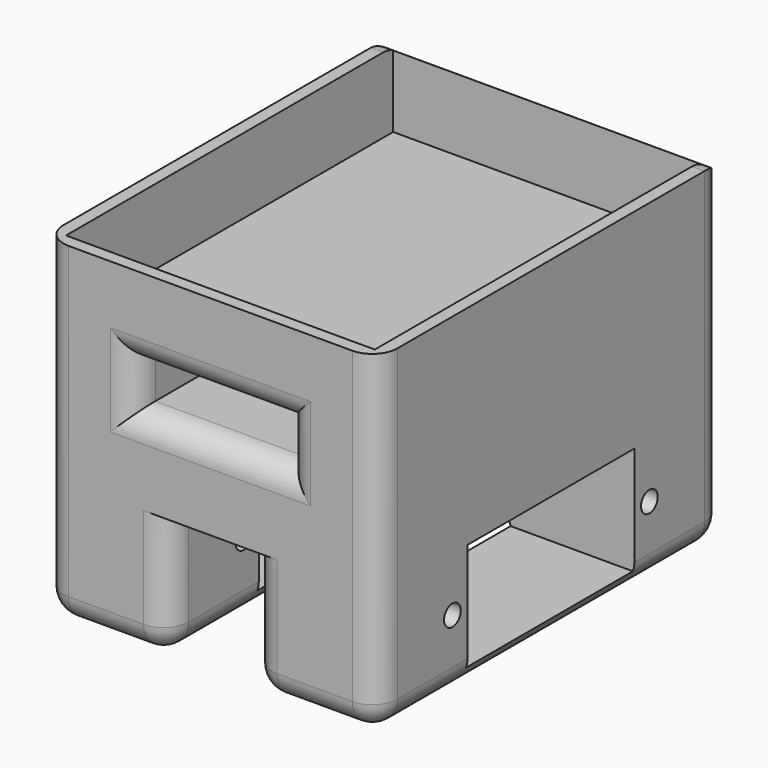
from build123d import *

# Parameters (mm, degrees)
F0_W           = 40
F0_H           = 52
F1_DEPTH       = 40
F2_W           = 25
F2_H           = 13
F2_R           = 1.25
F3_DEPTH       = 40.001
F4_W           = 10
F4_H           = 52
F5_DEPTH       = 15
F6_W           = 25
F6_H           = 6
F7_DEPTH       = 42
F8_W           = 18
F8_H           = 5
F9_DEPTH       = 42
F10_W          = 37
F10_H          = 49
F11_DEPTH      = 9
F12_T1_DEPTH   = 37
F12_T3_DEPTH   = 25
F12_T5_DEPTH   = 9
F12_T7_DEPTH   = 12
F12_T9_DEPTH   = 40
F12_T11_DEPTH  = 10
F12_T13_DEPTH  = 9
F12_T15_DEPTH  = 6
F12_T17_DEPTH  = 5
F12_T19_DEPTH  = 18
F12_T21_DEPTH  = 46
F12_S25_W      = 3.06
F12_S25_H      = 3.06
F12_T26_DEPTH  = 3.06
F12_S31_W      = 3.06
F12_S31_H      = 3.06
F12_T32_DEPTH  = 3.06
F12_S37_W      = 3.06
F12_S37_H      = 3.06
F12_T38_DEPTH  = 3.06
F12_S43_W      = 3.06
F12_S43_H      = 3.06
F12_T44_DEPTH  = 3.06
F12_S49_W      = 3.06
F12_S49_H      = 3.06
F12_T50_DEPTH  = 3.06
F12_S55_W      = 3.06
F12_S55_H      = 3.06
F12_T56_DEPTH  = 3.06
F12_S61_W      = 3.06
F12_S61_H      = 3.06
F12_T62_DEPTH  = 3.06
F12_S67_W      = 3.06
F12_S67_H      = 3.06
F12_T68_DEPTH  = 3.06
F12_T75_DEPTH  = 47.5
F12_T79_DEPTH  = 44.5
F12_T86_DEPTH  = 44.5
F12_T90_DEPTH  = 47.5
F12_T97_DEPTH  = 32.5
F12_T101_DEPTH = 13.5
F12_T108_DEPTH = 13.5
F12_T112_DEPTH = 32.5
F12_T119_DEPTH = 19.5
F12_T123_DEPTH = 17.5
F12_T130_DEPTH = 17.5
F12_T134_DEPTH = 19.5
F12_T141_DEPTH = 13.5
F12_T145_DEPTH = 32.5
F12_T152_DEPTH = 13.5
F12_T156_DEPTH = 32.5
F12_T163_DEPTH = 12.5
F12_T167_DEPTH = 25.5
F12_T174_DEPTH = 25.5
F12_T178_DEPTH = 12.5
F12_T185_DEPTH = 12.5
F12_T189_DEPTH = 25.5
F12_T196_DEPTH = 12.5
F12_T200_DEPTH = 25.5


# Not quite as in the source:
# - a fillet or chamfer that OpenCascade refuses, or shapes differently, is made with other operations: its cross-section is extruded or revolved along the edge and cut away or added


with BuildPart() as f1:
    # F0 (on Top) → F1 (new body)
    with BuildSketch(Plane.XY):
        with Locations((9.9251037464, 5.5336094776)):
            Rectangle(F0_W, F0_H)
    extrude(amount=F1_DEPTH)

    # F2 (on face) → F3 (cut, through all)
    with BuildSketch(Plane.YZ.offset(29.9251037464)):
        with Locations((5.5336094776, 8.5)):
            Rectangle(F2_W, F2_H)
        with Locations((-9.2163905224, 8.5)):
            Circle(F2_R)
        with Locations((20.2836094776, 8.5)):
            Circle(F2_R)
    extrude(amount=-F3_DEPTH, mode=Mode.SUBTRACT)

    # F4 (on face) → F5 (cut)
    with BuildSketch(Plane(origin=(0, 0, 0), x_dir=(1, 0, 0), z_dir=(0, 0, -1))):
        with Locations((9.9251037464, -5.5336094776)):
            Rectangle(F4_W, F4_H)
    extrude(amount=-F5_DEPTH, mode=Mode.SUBTRACT)

    # F6 (on face) → F7 (cut)
    with BuildSketch(Plane(origin=(0, 31.5336094776, 0), x_dir=(-1, 0, 0), z_dir=(0, 1, 0))):
        with Locations((-9.9251037464, 20)):
            Rectangle(F6_W, F6_H)
    extrude(amount=-F7_DEPTH, mode=Mode.SUBTRACT)

    # F8 (on face) → F9 (cut)
    with BuildSketch(Plane.XZ.offset(20.4663905224)):
        with Locations((9.9251037464, 27.5)):
            Rectangle(F8_W, F8_H)
    extrude(amount=-F9_DEPTH, mode=Mode.SUBTRACT)

    # F10 (on face) → F11 (cut)
    with BuildSketch(Plane.XY.offset(40)):
        with Locations((9.9251037464, 5.5336094776)):
            Rectangle(F10_W, F10_H)
    extrude(amount=-F11_DEPTH, mode=Mode.SUBTRACT)

    # F12: fillet of radius 3 on 26 edges, made by hand

    # F12_s2 → F12_t1 (cut)
    with BuildSketch(Plane.XY.offset(3)):
        with BuildLine():
            ThreePointArc((-10.0748962536, -17.4663905224), (-9.1962165972, -19.587710866), (-7.0748962536, -20.4663905224))
            Line((-7.0748962536, -20.4663905224), (-7.0748962536, -20.5263905224))
            Line((-7.0748962536, -20.5263905224), (-10.1348962536, -20.5263905224))
            Line((-10.1348962536, -20.5263905224), (-10.1348962536, -17.4663905224))
            Line((-10.1348962536, -17.4663905224), (-10.0748962536, -17.4663905224))
        make_face()
        with BuildLine():
            ThreePointArc((29.9251037464, -17.4663905224), (29.0464240899, -19.587710866), (26.9251037464, -20.4663905224))
            Line((26.9251037464, -20.4663905224), (26.9251037464, -20.5263905224))
            Line((26.9251037464, -20.5263905224), (29.9851037464, -20.5263905224))
            Line((29.9851037464, -20.5263905224), (29.9851037464, -17.4663905224))
            Line((29.9851037464, -17.4663905224), (29.9251037464, -17.4663905224))
        make_face()
        with BuildLine():
            ThreePointArc((-7.0748962536, 31.5336094776), (-9.1962165972, 30.6549298212), (-10.0748962536, 28.5336094776))
            Line((-10.0748962536, 28.5336094776), (-10.1348962536, 28.5336094776))
            Line((-10.1348962536, 28.5336094776), (-10.1348962536, 31.5936094776))
            Line((-10.1348962536, 31.5936094776), (-7.0748962536, 31.5936094776))
            Line((-7.0748962536, 31.5936094776), (-7.0748962536, 31.5336094776))
        make_face()
        with BuildLine():
            ThreePointArc((26.9251037464, 31.5336094776), (29.0464240899, 30.6549298212), (29.9251037464, 28.5336094776))
            Line((29.9251037464, 28.5336094776), (29.9851037464, 28.5336094776))
            Line((29.9851037464, 28.5336094776), (29.9851037464, 31.5936094776))
            Line((29.9851037464, 31.5936094776), (26.9251037464, 31.5936094776))
            Line((26.9251037464, 31.5936094776), (26.9251037464, 31.5336094776))
        make_face()
    extrude(amount=F12_T1_DEPTH, mode=Mode.SUBTRACT)

    # F12_s4 → F12_t3 (cut)
    with BuildSketch(Plane.YZ.offset(-2.5748962536)):
        with BuildLine():
            ThreePointArc((31.5336094776, 14), (30.6549298212, 16.1213203436), (28.5336094776, 17))
            Line((28.5336094776, 17), (28.5336094776, 17.06))
            Line((28.5336094776, 17.06), (31.5936094776, 17.06))
            Line((31.5936094776, 17.06), (31.5936094776, 14))
            Line((31.5936094776, 14), (31.5336094776, 14))
        make_face()
        with BuildLine():
            ThreePointArc((31.5336094776, 26), (30.6549298212, 23.8786796564), (28.5336094776, 23))
            Line((28.5336094776, 23), (28.5336094776, 22.94))
            Line((28.5336094776, 22.94), (31.5936094776, 22.94))
            Line((31.5936094776, 22.94), (31.5936094776, 26))
            Line((31.5936094776, 26), (31.5336094776, 26))
        make_face()
    extrude(amount=F12_T3_DEPTH, mode=Mode.SUBTRACT)

    # F12_s6 → F12_t5 (cut)
    with BuildSketch(Plane.YZ.offset(17.9251037464)):
        with BuildLine():
            ThreePointArc((31.5336094776, 3), (30.6549298212, 0.8786796564), (28.5336094776, 0))
            Line((28.5336094776, 0), (28.5336094776, -0.06))
            Line((28.5336094776, -0.06), (31.5936094776, -0.06))
            Line((31.5936094776, -0.06), (31.5936094776, 3))
            Line((31.5936094776, 3), (31.5336094776, 3))
        make_face()
        with BuildLine():
            ThreePointArc((-17.4663905224, 0), (-19.587710866, 0.8786796564), (-20.4663905224, 3))
            Line((-20.4663905224, 3), (-20.5263905224, 3))
            Line((-20.5263905224, 3), (-20.5263905224, -0.06))
            Line((-20.5263905224, -0.06), (-17.4663905224, -0.06))
            Line((-17.4663905224, -0.06), (-17.4663905224, 0))
        make_face()
    extrude(amount=F12_T5_DEPTH, mode=Mode.SUBTRACT)

    # F12_s8 → F12_t7 (cut)
    with BuildSketch(Plane.XY.offset(3)):
        with BuildLine():
            ThreePointArc((17.9251037464, 31.5336094776), (15.8037834028, 30.6549298212), (14.9251037464, 28.5336094776))
            Line((14.9251037464, 28.5336094776), (14.8651037464, 28.5336094776))
            Line((14.8651037464, 28.5336094776), (14.8651037464, 31.5936094776))
            Line((14.8651037464, 31.5936094776), (17.9251037464, 31.5936094776))
            Line((17.9251037464, 31.5936094776), (17.9251037464, 31.5336094776))
        make_face()
        with BuildLine():
            ThreePointArc((1.9251037464, 31.5336094776), (4.0464240899, 30.6549298212), (4.9251037464, 28.5336094776))
            Line((4.9251037464, 28.5336094776), (4.9851037464, 28.5336094776))
            Line((4.9851037464, 28.5336094776), (4.9851037464, 31.5936094776))
            Line((4.9851037464, 31.5936094776), (1.9251037464, 31.5936094776))
            Line((1.9251037464, 31.5936094776), (1.9251037464, 31.5336094776))
        make_face()
        with BuildLine():
            ThreePointArc((4.9251037464, -17.4663905224), (4.0464240899, -19.587710866), (1.9251037464, -20.4663905224))
            Line((1.9251037464, -20.4663905224), (1.9251037464, -20.5263905224))
            Line((1.9251037464, -20.5263905224), (4.9851037464, -20.5263905224))
            Line((4.9851037464, -20.5263905224), (4.9851037464, -17.4663905224))
            Line((4.9851037464, -17.4663905224), (4.9251037464, -17.4663905224))
        make_face()
        with BuildLine():
            ThreePointArc((14.9251037464, -17.4663905224), (15.8037834028, -19.587710866), (17.9251037464, -20.4663905224))
            Line((17.9251037464, -20.4663905224), (17.9251037464, -20.5263905224))
            Line((17.9251037464, -20.5263905224), (14.8651037464, -20.5263905224))
            Line((14.8651037464, -20.5263905224), (14.8651037464, -17.4663905224))
            Line((14.8651037464, -17.4663905224), (14.9251037464, -17.4663905224))
        make_face()
    extrude(amount=F12_T7_DEPTH, mode=Mode.SUBTRACT)

    # F12_s10 → F12_t9 (cut)
    with BuildSketch(Plane.YZ.offset(-10.0748962536)):
        with BuildLine():
            ThreePointArc((31.5336094776, 37), (30.6549298212, 39.1213203436), (28.5336094776, 40))
            Line((28.5336094776, 40), (28.5336094776, 40.06))
            Line((28.5336094776, 40.06), (31.5936094776, 40.06))
            Line((31.5936094776, 40.06), (31.5936094776, 37))
            Line((31.5936094776, 37), (31.5336094776, 37))
        make_face()
    extrude(amount=F12_T9_DEPTH, mode=Mode.SUBTRACT)

    # F12_s12 → F12_t11 (cut)
    with BuildSketch(Plane.YZ.offset(4.9251037464)):
        with BuildLine():
            ThreePointArc((31.5336094776, 18), (30.6549298212, 15.8786796564), (28.5336094776, 15))
            Line((28.5336094776, 15), (28.5336094776, 14.94))
            Line((28.5336094776, 14.94), (31.5936094776, 14.94))
            Line((31.5936094776, 14.94), (31.5936094776, 18))
            Line((31.5936094776, 18), (31.5336094776, 18))
        make_face()
    extrude(amount=F12_T11_DEPTH, mode=Mode.SUBTRACT)

    # F12_s14 → F12_t13 (cut)
    with BuildSketch(Plane.YZ.offset(-7.0748962536)):
        with BuildLine():
            ThreePointArc((31.5336094776, 3), (30.6549298212, 0.8786796564), (28.5336094776, 0))
            Line((28.5336094776, 0), (28.5336094776, -0.06))
            Line((28.5336094776, -0.06), (31.5936094776, -0.06))
            Line((31.5936094776, -0.06), (31.5936094776, 3))
            Line((31.5936094776, 3), (31.5336094776, 3))
        make_face()
        with BuildLine():
            ThreePointArc((-17.4663905224, 0), (-19.587710866, 0.8786796564), (-20.4663905224, 3))
            Line((-20.4663905224, 3), (-20.5263905224, 3))
            Line((-20.5263905224, 3), (-20.5263905224, -0.06))
            Line((-20.5263905224, -0.06), (-17.4663905224, -0.06))
            Line((-17.4663905224, -0.06), (-17.4663905224, 0))
        make_face()
    extrude(amount=F12_T13_DEPTH, mode=Mode.SUBTRACT)

    # F12_s16 → F12_t15 (cut)
    with BuildSketch(Plane.XY.offset(17)):
        with BuildLine():
            ThreePointArc((-5.5748962536, 31.5336094776), (-3.4535759101, 30.6549298212), (-2.5748962536, 28.5336094776))
            Line((-2.5748962536, 28.5336094776), (-2.5148962536, 28.5336094776))
            Line((-2.5148962536, 28.5336094776), (-2.5148962536, 31.5936094776))
            Line((-2.5148962536, 31.5936094776), (-5.5748962536, 31.5936094776))
            Line((-5.5748962536, 31.5936094776), (-5.5748962536, 31.5336094776))
        make_face()
        with BuildLine():
            ThreePointArc((25.4251037464, 31.5336094776), (23.3037834028, 30.6549298212), (22.4251037464, 28.5336094776))
            Line((22.4251037464, 28.5336094776), (22.3651037464, 28.5336094776))
            Line((22.3651037464, 28.5336094776), (22.3651037464, 31.5936094776))
            Line((22.3651037464, 31.5936094776), (25.4251037464, 31.5936094776))
            Line((25.4251037464, 31.5936094776), (25.4251037464, 31.5336094776))
        make_face()
    extrude(amount=F12_T15_DEPTH, mode=Mode.SUBTRACT)

    # F12_s18 → F12_t17 (cut)
    with BuildSketch(Plane.XY.offset(25)):
        with BuildLine():
            ThreePointArc((21.9251037464, -20.4663905224), (19.8037834028, -19.587710866), (18.9251037464, -17.4663905224))
            Line((18.9251037464, -17.4663905224), (18.8651037464, -17.4663905224))
            Line((18.8651037464, -17.4663905224), (18.8651037464, -20.5263905224))
            Line((18.8651037464, -20.5263905224), (21.9251037464, -20.5263905224))
            Line((21.9251037464, -20.5263905224), (21.9251037464, -20.4663905224))
        make_face()
        with BuildLine():
            ThreePointArc((-2.0748962536, -20.4663905224), (0.0464240899, -19.587710866), (0.9251037464, -17.4663905224))
            Line((0.9251037464, -17.4663905224), (0.9851037464, -17.4663905224))
            Line((0.9851037464, -17.4663905224), (0.9851037464, -20.5263905224))
            Line((0.9851037464, -20.5263905224), (-2.0748962536, -20.5263905224))
            Line((-2.0748962536, -20.5263905224), (-2.0748962536, -20.4663905224))
        make_face()
    extrude(amount=F12_T17_DEPTH, mode=Mode.SUBTRACT)

    # F12_s20 → F12_t19 (cut)
    with BuildSketch(Plane.YZ.offset(0.9251037464)):
        with BuildLine():
            ThreePointArc((-20.4663905224, 33), (-19.587710866, 30.8786796564), (-17.4663905224, 30))
            Line((-17.4663905224, 30), (-17.4663905224, 29.94))
            Line((-17.4663905224, 29.94), (-20.5263905224, 29.94))
            Line((-20.5263905224, 29.94), (-20.5263905224, 33))
            Line((-20.5263905224, 33), (-20.4663905224, 33))
        make_face()
        with BuildLine():
            ThreePointArc((-20.4663905224, 22), (-19.587710866, 24.1213203436), (-17.4663905224, 25))
            Line((-17.4663905224, 25), (-17.4663905224, 25.06))
            Line((-17.4663905224, 25.06), (-20.5263905224, 25.06))
            Line((-20.5263905224, 25.06), (-20.5263905224, 22))
            Line((-20.5263905224, 22), (-20.4663905224, 22))
        make_face()
    extrude(amount=F12_T19_DEPTH, mode=Mode.SUBTRACT)

    # F12_s22 → F12_t21 (cut)
    with BuildSketch(Plane.XZ.offset(-28.5336094776)):
        with BuildLine():
            ThreePointArc((-10.0748962536, 3), (-9.1962165972, 0.8786796564), (-7.0748962536, 0))
            Line((-7.0748962536, 0), (-7.0748962536, -0.06))
            Line((-7.0748962536, -0.06), (-10.1348962536, -0.06))
            Line((-10.1348962536, -0.06), (-10.1348962536, 3))
            Line((-10.1348962536, 3), (-10.0748962536, 3))
        make_face()
        with BuildLine():
            ThreePointArc((26.9251037464, 0), (29.0464240899, 0.8786796564), (29.9251037464, 3))
            Line((29.9251037464, 3), (29.9851037464, 3))
            Line((29.9851037464, 3), (29.9851037464, -0.06))
            Line((29.9851037464, -0.06), (26.9251037464, -0.06))
            Line((26.9251037464, -0.06), (26.9251037464, 0))
        make_face()
        with BuildLine():
            ThreePointArc((4.9251037464, 3), (4.0464240899, 0.8786796564), (1.9251037464, 0))
            Line((1.9251037464, 0), (1.9251037464, -0.06))
            Line((1.9251037464, -0.06), (4.9851037464, -0.06))
            Line((4.9851037464, -0.06), (4.9851037464, 3))
            Line((4.9851037464, 3), (4.9251037464, 3))
        make_face()
        with BuildLine():
            ThreePointArc((17.9251037464, 0), (15.8037834028, 0.8786796564), (14.9251037464, 3))
            Line((14.9251037464, 3), (14.8651037464, 3))
            Line((14.8651037464, 3), (14.8651037464, -0.06))
            Line((14.8651037464, -0.06), (17.9251037464, -0.06))
            Line((17.9251037464, -0.06), (17.9251037464, 0))
        make_face()
    extrude(amount=F12_T21_DEPTH, mode=Mode.SUBTRACT)


with BuildPart() as f12_tool24:
    # F12_s25 → F12_t26 (new body)
    with BuildSketch(Plane.XY.offset(3)):
        with Locations((-8.6048962536, -18.9963905224)):
            Rectangle(F12_S25_W, F12_S25_H)
    extrude(amount=-F12_T26_DEPTH)

    # F12_s27 → F12_t28 (revolve, cut)
    with BuildSketch(Plane(origin=(-7.0748962536, -17.4663905224, 3), x_dir=(0.7071067812, 0.7071067812, 0), z_dir=(-0.7071067812, 0.7071067812, 0))):
        with BuildLine():
            ThreePointArc((0, -3), (3, 0), (0, 3))
            Line((0, 3), (0, -3))
        make_face()
    revolve(axis=Axis((-7.0748962536, -17.4663905224, 3), (0, 0, -1)), mode=Mode.SUBTRACT)


with BuildPart() as f1_1:
    add(f1.part)

    # F12_t23: cut F12_tool24
    add(f12_tool24.part, mode=Mode.SUBTRACT)


with BuildPart() as f12_tool30:
    # F12_s31 → F12_t32 (new body)
    with BuildSketch(Plane.XY.offset(3)):
        with Locations((28.4551037464, -18.9963905224)):
            Rectangle(F12_S31_W, F12_S31_H)
    extrude(amount=-F12_T32_DEPTH)

    # F12_s33 → F12_t34 (revolve, cut)
    with BuildSketch(Plane(origin=(26.9251037464, -17.4663905224, 3), x_dir=(-0.7071067812, 0.7071067812, 0), z_dir=(-0.7071067812, -0.7071067812, 0))):
        with BuildLine():
            ThreePointArc((0, -3), (3, 0), (0, 3))
            Line((0, 3), (0, -3))
        make_face()
    revolve(axis=Axis((26.9251037464, -17.4663905224, 3), (0, 0, -1)), mode=Mode.SUBTRACT)


with BuildPart() as f1_2:
    add(f1_1.part)

    # F12_t29: cut F12_tool30
    add(f12_tool30.part, mode=Mode.SUBTRACT)


with BuildPart() as f12_tool36:
    # F12_s37 → F12_t38 (new body)
    with BuildSketch(Plane.XZ.offset(-28.5336094776)):
        with Locations((-8.6048962536, 1.47)):
            Rectangle(F12_S37_W, F12_S37_H)
    extrude(amount=-F12_T38_DEPTH)

    # F12_s39 → F12_t40 (revolve, cut)
    with BuildSketch(Plane(origin=(-7.0748962536, 28.5336094776, 3), x_dir=(0.7071067812, 0, 0.7071067812), z_dir=(-0.7071067812, 0, 0.7071067812))):
        with BuildLine():
            ThreePointArc((0, -3), (3, 0), (0, 3))
            Line((0, 3), (0, -3))
        make_face()
    revolve(axis=Axis((-7.0748962536, 28.5336094776, 3), (0, 1, 0)), mode=Mode.SUBTRACT)


with BuildPart() as f1_3:
    add(f1_2.part)

    # F12_t35: cut F12_tool36
    add(f12_tool36.part, mode=Mode.SUBTRACT)


with BuildPart() as f12_tool42:
    # F12_s43 → F12_t44 (new body)
    with BuildSketch(Plane.XZ.offset(-28.5336094776)):
        with Locations((28.4551037464, 1.47)):
            Rectangle(F12_S43_W, F12_S43_H)
    extrude(amount=-F12_T44_DEPTH)

    # F12_s45 → F12_t46 (revolve, cut)
    with BuildSketch(Plane(origin=(26.9251037464, 28.5336094776, 3), x_dir=(-0.7071067812, 0, 0.7071067812), z_dir=(-0.7071067812, 0, -0.7071067812))):
        with BuildLine():
            ThreePointArc((0, -3), (3, 0), (0, 3))
            Line((0, 3), (0, -3))
        make_face()
    revolve(axis=Axis((26.9251037464, 28.5336094776, 3), (0, 1, 0)), mode=Mode.SUBTRACT)


with BuildPart() as f1_4:
    add(f1_3.part)

    # F12_t41: cut F12_tool42
    add(f12_tool42.part, mode=Mode.SUBTRACT)


with BuildPart() as f12_tool48:
    # F12_s49 → F12_t50 (new body)
    with BuildSketch(Plane.XZ.offset(-28.5336094776)):
        with Locations((16.3951037464, 1.47)):
            Rectangle(F12_S49_W, F12_S49_H)
    extrude(amount=-F12_T50_DEPTH)

    # F12_s51 → F12_t52 (revolve, cut)
    with BuildSketch(Plane(origin=(17.9251037464, 28.5336094776, 3), x_dir=(0.7071067812, 0, 0.7071067812), z_dir=(-0.7071067812, 0, 0.7071067812))):
        with BuildLine():
            ThreePointArc((0, -3), (3, 0), (0, 3))
            Line((0, 3), (0, -3))
        make_face()
    revolve(axis=Axis((17.9251037464, 28.5336094776, 3), (0, 1, 0)), mode=Mode.SUBTRACT)


with BuildPart() as f1_5:
    add(f1_4.part)

    # F12_t47: cut F12_tool48
    add(f12_tool48.part, mode=Mode.SUBTRACT)


with BuildPart() as f12_tool54:
    # F12_s55 → F12_t56 (new body)
    with BuildSketch(Plane.XZ.offset(-28.5336094776)):
        with Locations((3.4551037464, 1.47)):
            Rectangle(F12_S55_W, F12_S55_H)
    extrude(amount=-F12_T56_DEPTH)

    # F12_s57 → F12_t58 (revolve, cut)
    with BuildSketch(Plane(origin=(1.9251037464, 28.5336094776, 3), x_dir=(-0.7071067812, 0, 0.7071067812), z_dir=(-0.7071067812, 0, -0.7071067812))):
        with BuildLine():
            ThreePointArc((0, -3), (3, 0), (0, 3))
            Line((0, 3), (0, -3))
        make_face()
    revolve(axis=Axis((1.9251037464, 28.5336094776, 3), (0, 1, 0)), mode=Mode.SUBTRACT)


with BuildPart() as f1_6:
    add(f1_5.part)

    # F12_t53: cut F12_tool54
    add(f12_tool54.part, mode=Mode.SUBTRACT)


with BuildPart() as f12_tool60:
    # F12_s61 → F12_t62 (new body)
    with BuildSketch(Plane.XY.offset(3)):
        with Locations((16.3951037464, -18.9963905224)):
            Rectangle(F12_S61_W, F12_S61_H)
    extrude(amount=-F12_T62_DEPTH)

    # F12_s63 → F12_t64 (revolve, cut)
    with BuildSketch(Plane(origin=(17.9251037464, -17.4663905224, 3), x_dir=(0.7071067812, 0.7071067812, 0), z_dir=(-0.7071067812, 0.7071067812, 0))):
        with BuildLine():
            ThreePointArc((0, -3), (3, 0), (0, 3))
            Line((0, 3), (0, -3))
        make_face()
    revolve(axis=Axis((17.9251037464, -17.4663905224, 3), (0, 0, -1)), mode=Mode.SUBTRACT)


with BuildPart() as f1_7:
    add(f1_6.part)

    # F12_t59: cut F12_tool60
    add(f12_tool60.part, mode=Mode.SUBTRACT)


with BuildPart() as f12_tool66:
    # F12_s67 → F12_t68 (new body)
    with BuildSketch(Plane.XY.offset(3)):
        with Locations((3.4551037464, -18.9963905224)):
            Rectangle(F12_S67_W, F12_S67_H)
    extrude(amount=-F12_T68_DEPTH)

    # F12_s69 → F12_t70 (revolve, cut)
    with BuildSketch(Plane(origin=(1.9251037464, -17.4663905224, 3), x_dir=(-0.7071067812, 0.7071067812, 0), z_dir=(-0.7071067812, -0.7071067812, 0))):
        with BuildLine():
            ThreePointArc((0, -3), (3, 0), (0, 3))
            Line((0, 3), (0, -3))
        make_face()
    revolve(axis=Axis((1.9251037464, -17.4663905224, 3), (0, 0, -1)), mode=Mode.SUBTRACT)


with BuildPart() as f1_8:
    add(f1_7.part)

    # F12_t65: cut F12_tool66
    add(f12_tool66.part, mode=Mode.SUBTRACT)


with BuildPart() as f12_tool73:
    # F12_s74 → F12_t75 (new body)
    with BuildSketch(Plane.YZ.offset(29.9251037464)):
        with BuildLine():
            ThreePointArc((31.5336094776, 37), (30.6549298212, 39.1213203436), (28.5336094776, 40))
            Line((28.5336094776, 40), (28.5336094776, 40.06))
            Line((28.5336094776, 40.06), (31.5936094776, 40.06))
            Line((31.5936094776, 40.06), (31.5936094776, 37))
            Line((31.5936094776, 37), (31.5336094776, 37))
        make_face()
    extrude(amount=-F12_T75_DEPTH)

    split(bisect_by=Plane.YZ.offset(-10.0748962536), keep=Keep.BOTTOM)


with BuildPart() as f12_tool77:
    # F12_s78 → F12_t79 (new body)
    with BuildSketch(Plane.XY.offset(3)):
        with BuildLine():
            ThreePointArc((-7.0748962536, 31.5336094776), (-9.1962165972, 30.6549298212), (-10.0748962536, 28.5336094776))
            Line((-10.0748962536, 28.5336094776), (-10.1348962536, 28.5336094776))
            Line((-10.1348962536, 28.5336094776), (-10.1348962536, 31.5936094776))
            Line((-10.1348962536, 31.5936094776), (-7.0748962536, 31.5936094776))
            Line((-7.0748962536, 31.5936094776), (-7.0748962536, 31.5336094776))
        make_face()
    extrude(amount=F12_T79_DEPTH)

    split(bisect_by=Plane.XY.offset(40), keep=Keep.TOP)


with BuildPart() as f12_tool73_1:
    add(f12_tool73.part)

    # F12_t81: intersect F12_tool77
    add(f12_tool77.part, mode=Mode.INTERSECT)


with BuildPart() as f1_9:
    add(f1_8.part)

    # F12_t71: cut F12_tool73
    add(f12_tool73_1.part, mode=Mode.SUBTRACT)


with BuildPart() as f12_tool84:
    # F12_s85 → F12_t86 (new body)
    with BuildSketch(Plane.XY.offset(3)):
        with BuildLine():
            ThreePointArc((26.9251037464, 31.5336094776), (29.0464240899, 30.6549298212), (29.9251037464, 28.5336094776))
            Line((29.9251037464, 28.5336094776), (29.9851037464, 28.5336094776))
            Line((29.9851037464, 28.5336094776), (29.9851037464, 31.5936094776))
            Line((29.9851037464, 31.5936094776), (26.9251037464, 31.5936094776))
            Line((26.9251037464, 31.5936094776), (26.9251037464, 31.5336094776))
        make_face()
    extrude(amount=F12_T86_DEPTH)

    split(bisect_by=Plane.XY.offset(40), keep=Keep.TOP)


with BuildPart() as f12_tool88:
    # F12_s89 → F12_t90 (new body)
    with BuildSketch(Plane.YZ.offset(37.4251037464)):
        with BuildLine():
            ThreePointArc((31.5336094776, 37), (30.6549298212, 39.1213203436), (28.5336094776, 40))
            Line((28.5336094776, 40), (28.5336094776, 40.06))
            Line((28.5336094776, 40.06), (31.5936094776, 40.06))
            Line((31.5936094776, 40.06), (31.5936094776, 37))
            Line((31.5936094776, 37), (31.5336094776, 37))
        make_face()
    extrude(amount=-F12_T90_DEPTH)

    split(bisect_by=Plane.YZ.offset(29.9251037464), keep=Keep.TOP)


with BuildPart() as f12_tool84_1:
    add(f12_tool84.part)

    # F12_t92: intersect F12_tool88
    add(f12_tool88.part, mode=Mode.INTERSECT)


with BuildPart() as f1_10:
    add(f1_9.part)

    # F12_t82: cut F12_tool84
    add(f12_tool84_1.part, mode=Mode.SUBTRACT)


with BuildPart() as f12_tool95:
    # F12_s96 → F12_t97 (new body)
    with BuildSketch(Plane.YZ.offset(29.9251037464)):
        with BuildLine():
            ThreePointArc((31.5336094776, 14), (30.6549298212, 16.1213203436), (28.5336094776, 17))
            Line((28.5336094776, 17), (28.5336094776, 17.06))
            Line((28.5336094776, 17.06), (31.5936094776, 17.06))
            Line((31.5936094776, 17.06), (31.5936094776, 14))
            Line((31.5936094776, 14), (31.5336094776, 14))
        make_face()
    extrude(amount=-F12_T97_DEPTH)

    split(bisect_by=Plane.YZ.offset(22.4251037464), keep=Keep.TOP)


with BuildPart() as f12_tool99:
    # F12_s100 → F12_t101 (new body)
    with BuildSketch(Plane.XY.offset(23)):
        with BuildLine():
            ThreePointArc((25.4251037464, 31.5336094776), (23.3037834028, 30.6549298212), (22.4251037464, 28.5336094776))
            Line((22.4251037464, 28.5336094776), (22.3651037464, 28.5336094776))
            Line((22.3651037464, 28.5336094776), (22.3651037464, 31.5936094776))
            Line((22.3651037464, 31.5936094776), (25.4251037464, 31.5936094776))
            Line((25.4251037464, 31.5936094776), (25.4251037464, 31.5336094776))
        make_face()
    extrude(amount=-F12_T101_DEPTH)

    split(bisect_by=Plane.XY.offset(17), keep=Keep.BOTTOM)


with BuildPart() as f12_tool95_1:
    add(f12_tool95.part)

    # F12_t103: intersect F12_tool99
    add(f12_tool99.part, mode=Mode.INTERSECT)


with BuildPart() as f1_11:
    add(f1_10.part)

    # F12_t93: cut F12_tool95
    add(f12_tool95_1.part, mode=Mode.SUBTRACT)


with BuildPart() as f12_tool106:
    # F12_s107 → F12_t108 (new body)
    with BuildSketch(Plane.XY.offset(9.5)):
        with BuildLine():
            ThreePointArc((-5.5748962536, 31.5336094776), (-3.4535759101, 30.6549298212), (-2.5748962536, 28.5336094776))
            Line((-2.5748962536, 28.5336094776), (-2.5148962536, 28.5336094776))
            Line((-2.5148962536, 28.5336094776), (-2.5148962536, 31.5936094776))
            Line((-2.5148962536, 31.5936094776), (-5.5748962536, 31.5936094776))
            Line((-5.5748962536, 31.5936094776), (-5.5748962536, 31.5336094776))
        make_face()
    extrude(amount=F12_T108_DEPTH)

    split(bisect_by=Plane.XY.offset(17), keep=Keep.BOTTOM)


with BuildPart() as f12_tool110:
    # F12_s111 → F12_t112 (new body)
    with BuildSketch(Plane.YZ.offset(22.4251037464)):
        with BuildLine():
            ThreePointArc((31.5336094776, 14), (30.6549298212, 16.1213203436), (28.5336094776, 17))
            Line((28.5336094776, 17), (28.5336094776, 17.06))
            Line((28.5336094776, 17.06), (31.5936094776, 17.06))
            Line((31.5936094776, 17.06), (31.5936094776, 14))
            Line((31.5936094776, 14), (31.5336094776, 14))
        make_face()
    extrude(amount=-F12_T112_DEPTH)

    split(bisect_by=Plane.YZ.offset(-2.5748962536), keep=Keep.BOTTOM)


with BuildPart() as f12_tool106_1:
    add(f12_tool106.part)

    # F12_t114: intersect F12_tool110
    add(f12_tool110.part, mode=Mode.INTERSECT)


with BuildPart() as f1_12:
    add(f1_11.part)

    # F12_t104: cut F12_tool106
    add(f12_tool106_1.part, mode=Mode.SUBTRACT)


with BuildPart() as f12_tool117:
    # F12_s118 → F12_t119 (new body)
    with BuildSketch(Plane.XY.offset(3)):
        with BuildLine():
            ThreePointArc((17.9251037464, 31.5336094776), (15.8037834028, 30.6549298212), (14.9251037464, 28.5336094776))
            Line((14.9251037464, 28.5336094776), (14.8651037464, 28.5336094776))
            Line((14.8651037464, 28.5336094776), (14.8651037464, 31.5936094776))
            Line((14.8651037464, 31.5936094776), (17.9251037464, 31.5936094776))
            Line((17.9251037464, 31.5936094776), (17.9251037464, 31.5336094776))
        make_face()
    extrude(amount=F12_T119_DEPTH)

    split(bisect_by=Plane.XY.offset(15), keep=Keep.TOP)


with BuildPart() as f12_tool121:
    # F12_s122 → F12_t123 (new body)
    with BuildSketch(Plane.YZ.offset(4.9251037464)):
        with BuildLine():
            ThreePointArc((31.5336094776, 18), (30.6549298212, 15.8786796564), (28.5336094776, 15))
            Line((28.5336094776, 15), (28.5336094776, 14.94))
            Line((28.5336094776, 14.94), (31.5936094776, 14.94))
            Line((31.5936094776, 14.94), (31.5936094776, 18))
            Line((31.5936094776, 18), (31.5336094776, 18))
        make_face()
    extrude(amount=F12_T123_DEPTH)

    split(bisect_by=Plane.YZ.offset(14.9251037464), keep=Keep.TOP)


with BuildPart() as f12_tool117_1:
    add(f12_tool117.part)

    # F12_t125: intersect F12_tool121
    add(f12_tool121.part, mode=Mode.INTERSECT)


with BuildPart() as f1_13:
    add(f1_12.part)

    # F12_t115: cut F12_tool117
    add(f12_tool117_1.part, mode=Mode.SUBTRACT)


with BuildPart() as f12_tool128:
    # F12_s129 → F12_t130 (new body)
    with BuildSketch(Plane.YZ.offset(-2.5748962536)):
        with BuildLine():
            ThreePointArc((31.5336094776, 18), (30.6549298212, 15.8786796564), (28.5336094776, 15))
            Line((28.5336094776, 15), (28.5336094776, 14.94))
            Line((28.5336094776, 14.94), (31.5936094776, 14.94))
            Line((31.5936094776, 14.94), (31.5936094776, 18))
            Line((31.5936094776, 18), (31.5336094776, 18))
        make_face()
    extrude(amount=F12_T130_DEPTH)

    split(bisect_by=Plane.YZ.offset(4.9251037464), keep=Keep.BOTTOM)


with BuildPart() as f12_tool132:
    # F12_s133 → F12_t134 (new body)
    with BuildSketch(Plane.XY.offset(3)):
        with BuildLine():
            ThreePointArc((1.9251037464, 31.5336094776), (4.0464240899, 30.6549298212), (4.9251037464, 28.5336094776))
            Line((4.9251037464, 28.5336094776), (4.9851037464, 28.5336094776))
            Line((4.9851037464, 28.5336094776), (4.9851037464, 31.5936094776))
            Line((4.9851037464, 31.5936094776), (1.9251037464, 31.5936094776))
            Line((1.9251037464, 31.5936094776), (1.9251037464, 31.5336094776))
        make_face()
    extrude(amount=F12_T134_DEPTH)

    split(bisect_by=Plane.XY.offset(15), keep=Keep.TOP)


with BuildPart() as f12_tool128_1:
    add(f12_tool128.part)

    # F12_t136: intersect F12_tool132
    add(f12_tool132.part, mode=Mode.INTERSECT)


with BuildPart() as f1_14:
    add(f1_13.part)

    # F12_t126: cut F12_tool128
    add(f12_tool128_1.part, mode=Mode.SUBTRACT)


with BuildPart() as f12_tool139:
    # F12_s140 → F12_t141 (new body)
    with BuildSketch(Plane.XY.offset(17)):
        with BuildLine():
            ThreePointArc((-5.5748962536, 31.5336094776), (-3.4535759101, 30.6549298212), (-2.5748962536, 28.5336094776))
            Line((-2.5748962536, 28.5336094776), (-2.5148962536, 28.5336094776))
            Line((-2.5148962536, 28.5336094776), (-2.5148962536, 31.5936094776))
            Line((-2.5148962536, 31.5936094776), (-5.5748962536, 31.5936094776))
            Line((-5.5748962536, 31.5936094776), (-5.5748962536, 31.5336094776))
        make_face()
    extrude(amount=F12_T141_DEPTH)

    split(bisect_by=Plane.XY.offset(23), keep=Keep.TOP)


with BuildPart() as f12_tool143:
    # F12_s144 → F12_t145 (new body)
    with BuildSketch(Plane.YZ.offset(-10.0748962536)):
        with BuildLine():
            ThreePointArc((31.5336094776, 26), (30.6549298212, 23.8786796564), (28.5336094776, 23))
            Line((28.5336094776, 23), (28.5336094776, 22.94))
            Line((28.5336094776, 22.94), (31.5936094776, 22.94))
            Line((31.5936094776, 22.94), (31.5936094776, 26))
            Line((31.5936094776, 26), (31.5336094776, 26))
        make_face()
    extrude(amount=F12_T145_DEPTH)

    split(bisect_by=Plane.YZ.offset(-2.5748962536), keep=Keep.BOTTOM)


with BuildPart() as f12_tool139_1:
    add(f12_tool139.part)

    # F12_t147: intersect F12_tool143
    add(f12_tool143.part, mode=Mode.INTERSECT)


with BuildPart() as f1_15:
    add(f1_14.part)

    # F12_t137: cut F12_tool139
    add(f12_tool139_1.part, mode=Mode.SUBTRACT)


with BuildPart() as f12_tool150:
    # F12_s151 → F12_t152 (new body)
    with BuildSketch(Plane.XY.offset(30.5)):
        with BuildLine():
            ThreePointArc((25.4251037464, 31.5336094776), (23.3037834028, 30.6549298212), (22.4251037464, 28.5336094776))
            Line((22.4251037464, 28.5336094776), (22.3651037464, 28.5336094776))
            Line((22.3651037464, 28.5336094776), (22.3651037464, 31.5936094776))
            Line((22.3651037464, 31.5936094776), (25.4251037464, 31.5936094776))
            Line((25.4251037464, 31.5936094776), (25.4251037464, 31.5336094776))
        make_face()
    extrude(amount=-F12_T152_DEPTH)

    split(bisect_by=Plane.XY.offset(23), keep=Keep.TOP)


with BuildPart() as f12_tool154:
    # F12_s155 → F12_t156 (new body)
    with BuildSketch(Plane.YZ.offset(-2.5748962536)):
        with BuildLine():
            ThreePointArc((31.5336094776, 26), (30.6549298212, 23.8786796564), (28.5336094776, 23))
            Line((28.5336094776, 23), (28.5336094776, 22.94))
            Line((28.5336094776, 22.94), (31.5936094776, 22.94))
            Line((31.5936094776, 22.94), (31.5936094776, 26))
            Line((31.5936094776, 26), (31.5336094776, 26))
        make_face()
    extrude(amount=F12_T156_DEPTH)

    split(bisect_by=Plane.YZ.offset(22.4251037464), keep=Keep.TOP)


with BuildPart() as f12_tool150_1:
    add(f12_tool150.part)

    # F12_t158: intersect F12_tool154
    add(f12_tool154.part, mode=Mode.INTERSECT)


with BuildPart() as f1_16:
    add(f1_15.part)

    # F12_t148: cut F12_tool150
    add(f12_tool150_1.part, mode=Mode.SUBTRACT)


with BuildPart() as f12_tool161:
    # F12_s162 → F12_t163 (new body)
    with BuildSketch(Plane.XY.offset(17.5)):
        with BuildLine():
            ThreePointArc((21.9251037464, -20.4663905224), (19.8037834028, -19.587710866), (18.9251037464, -17.4663905224))
            Line((18.9251037464, -17.4663905224), (18.8651037464, -17.4663905224))
            Line((18.8651037464, -17.4663905224), (18.8651037464, -20.5263905224))
            Line((18.8651037464, -20.5263905224), (21.9251037464, -20.5263905224))
            Line((21.9251037464, -20.5263905224), (21.9251037464, -20.4663905224))
        make_face()
    extrude(amount=F12_T163_DEPTH)

    split(bisect_by=Plane.XY.offset(25), keep=Keep.BOTTOM)


with BuildPart() as f12_tool165:
    # F12_s166 → F12_t167 (new body)
    with BuildSketch(Plane.YZ.offset(0.9251037464)):
        with BuildLine():
            ThreePointArc((-20.4663905224, 22), (-19.587710866, 24.1213203436), (-17.4663905224, 25))
            Line((-17.4663905224, 25), (-17.4663905224, 25.06))
            Line((-17.4663905224, 25.06), (-20.5263905224, 25.06))
            Line((-20.5263905224, 25.06), (-20.5263905224, 22))
            Line((-20.5263905224, 22), (-20.4663905224, 22))
        make_face()
    extrude(amount=F12_T167_DEPTH)

    split(bisect_by=Plane.YZ.offset(18.9251037464), keep=Keep.TOP)


with BuildPart() as f12_tool161_1:
    add(f12_tool161.part)

    # F12_t169: intersect F12_tool165
    add(f12_tool165.part, mode=Mode.INTERSECT)


with BuildPart() as f1_17:
    add(f1_16.part)

    # F12_t159: cut F12_tool161
    add(f12_tool161_1.part, mode=Mode.SUBTRACT)


with BuildPart() as f12_tool172:
    # F12_s173 → F12_t174 (new body)
    with BuildSketch(Plane.YZ.offset(26.4251037464)):
        with BuildLine():
            ThreePointArc((-20.4663905224, 33), (-19.587710866, 30.8786796564), (-17.4663905224, 30))
            Line((-17.4663905224, 30), (-17.4663905224, 29.94))
            Line((-17.4663905224, 29.94), (-20.5263905224, 29.94))
            Line((-20.5263905224, 29.94), (-20.5263905224, 33))
            Line((-20.5263905224, 33), (-20.4663905224, 33))
        make_face()
    extrude(amount=-F12_T174_DEPTH)

    split(bisect_by=Plane.YZ.offset(18.9251037464), keep=Keep.TOP)


with BuildPart() as f12_tool176:
    # F12_s177 → F12_t178 (new body)
    with BuildSketch(Plane.XY.offset(25)):
        with BuildLine():
            ThreePointArc((21.9251037464, -20.4663905224), (19.8037834028, -19.587710866), (18.9251037464, -17.4663905224))
            Line((18.9251037464, -17.4663905224), (18.8651037464, -17.4663905224))
            Line((18.8651037464, -17.4663905224), (18.8651037464, -20.5263905224))
            Line((18.8651037464, -20.5263905224), (21.9251037464, -20.5263905224))
            Line((21.9251037464, -20.5263905224), (21.9251037464, -20.4663905224))
        make_face()
    extrude(amount=F12_T178_DEPTH)

    split(bisect_by=Plane.XY.offset(30), keep=Keep.TOP)


with BuildPart() as f12_tool172_1:
    add(f12_tool172.part)

    # F12_t180: intersect F12_tool176
    add(f12_tool176.part, mode=Mode.INTERSECT)


with BuildPart() as f1_18:
    add(f1_17.part)

    # F12_t170: cut F12_tool172
    add(f12_tool172_1.part, mode=Mode.SUBTRACT)


with BuildPart() as f12_tool183:
    # F12_s184 → F12_t185 (new body)
    with BuildSketch(Plane.XY.offset(37.5)):
        with BuildLine():
            ThreePointArc((-2.0748962536, -20.4663905224), (0.0464240899, -19.587710866), (0.9251037464, -17.4663905224))
            Line((0.9251037464, -17.4663905224), (0.9851037464, -17.4663905224))
            Line((0.9851037464, -17.4663905224), (0.9851037464, -20.5263905224))
            Line((0.9851037464, -20.5263905224), (-2.0748962536, -20.5263905224))
            Line((-2.0748962536, -20.5263905224), (-2.0748962536, -20.4663905224))
        make_face()
    extrude(amount=-F12_T185_DEPTH)

    split(bisect_by=Plane.XY.offset(30), keep=Keep.TOP)


with BuildPart() as f12_tool187:
    # F12_s188 → F12_t189 (new body)
    with BuildSketch(Plane.YZ.offset(18.9251037464)):
        with BuildLine():
            ThreePointArc((-20.4663905224, 33), (-19.587710866, 30.8786796564), (-17.4663905224, 30))
            Line((-17.4663905224, 30), (-17.4663905224, 29.94))
            Line((-17.4663905224, 29.94), (-20.5263905224, 29.94))
            Line((-20.5263905224, 29.94), (-20.5263905224, 33))
            Line((-20.5263905224, 33), (-20.4663905224, 33))
        make_face()
    extrude(amount=-F12_T189_DEPTH)

    split(bisect_by=Plane.YZ.offset(0.9251037464), keep=Keep.BOTTOM)


with BuildPart() as f12_tool183_1:
    add(f12_tool183.part)

    # F12_t191: intersect F12_tool187
    add(f12_tool187.part, mode=Mode.INTERSECT)


with BuildPart() as f1_19:
    add(f1_18.part)

    # F12_t181: cut F12_tool183
    add(f12_tool183_1.part, mode=Mode.SUBTRACT)


with BuildPart() as f12_tool194:
    # F12_s195 → F12_t196 (new body)
    with BuildSketch(Plane.XY.offset(30)):
        with BuildLine():
            ThreePointArc((-2.0748962536, -20.4663905224), (0.0464240899, -19.587710866), (0.9251037464, -17.4663905224))
            Line((0.9251037464, -17.4663905224), (0.9851037464, -17.4663905224))
            Line((0.9851037464, -17.4663905224), (0.9851037464, -20.5263905224))
            Line((0.9851037464, -20.5263905224), (-2.0748962536, -20.5263905224))
            Line((-2.0748962536, -20.5263905224), (-2.0748962536, -20.4663905224))
        make_face()
    extrude(amount=-F12_T196_DEPTH)

    split(bisect_by=Plane.XY.offset(25), keep=Keep.BOTTOM)


with BuildPart() as f12_tool198:
    # F12_s199 → F12_t200 (new body)
    with BuildSketch(Plane.YZ.offset(-6.5748962536)):
        with BuildLine():
            ThreePointArc((-20.4663905224, 22), (-19.587710866, 24.1213203436), (-17.4663905224, 25))
            Line((-17.4663905224, 25), (-17.4663905224, 25.06))
            Line((-17.4663905224, 25.06), (-20.5263905224, 25.06))
            Line((-20.5263905224, 25.06), (-20.5263905224, 22))
            Line((-20.5263905224, 22), (-20.4663905224, 22))
        make_face()
    extrude(amount=F12_T200_DEPTH)

    split(bisect_by=Plane.YZ.offset(0.9251037464), keep=Keep.BOTTOM)


with BuildPart() as f12_tool194_1:
    add(f12_tool194.part)

    # F12_t202: intersect F12_tool198
    add(f12_tool198.part, mode=Mode.INTERSECT)


with BuildPart() as f1_20:
    add(f1_19.part)

    # F12_t192: cut F12_tool194
    add(f12_tool194_1.part, mode=Mode.SUBTRACT)


solid = f1_20.part
